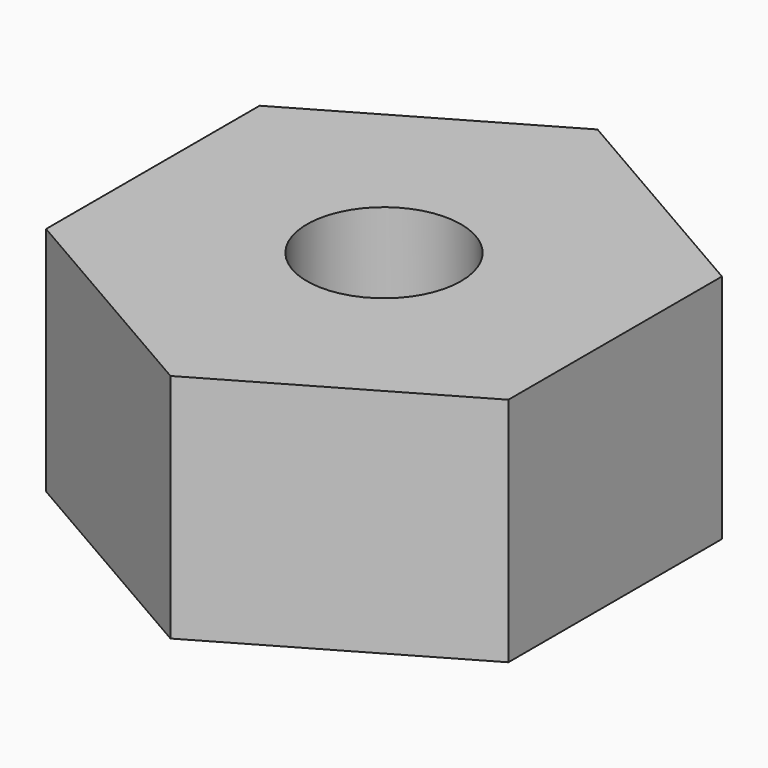
from build123d import *

# Parameters (mm, degrees)
F1_DEPTH = 4.7625
F2_R     = 1.5875
F3_DEPTH = 4.7635


# Not quite as in the source:
# - a feature names something its author has since deleted; it is built from what else it names


with BuildPart() as f1:
    # F0 (on Top) → F1 (new body)
    with BuildSketch(Plane.XY):
        Polygon((4.7625, -2.749630657), (4.7625, 2.749630657), (0, 5.499261314), (-4.7625, 2.749630657), (-4.7625, -2.749630657), (0, -5.499261314), align=None)
    extrude(amount=F1_DEPTH)

    # F2 (on face) → F3 (cut, through all)
    with BuildSketch(Plane.XY.offset(4.7625)):
        Circle(F2_R)
    extrude(amount=-F3_DEPTH, mode=Mode.SUBTRACT)


solid = f1.part
